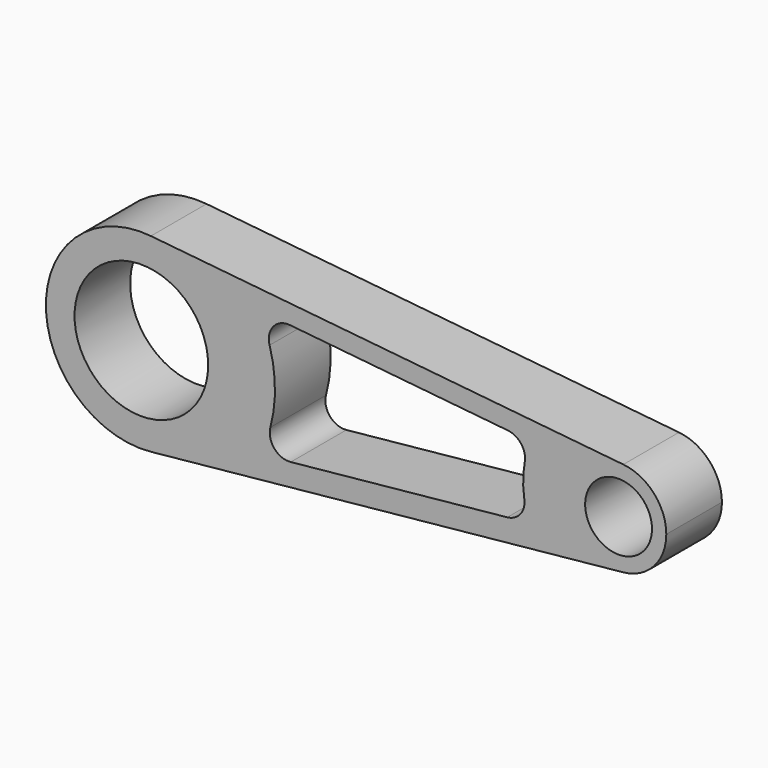
from build123d import *

# Parameters (mm, degrees)
F0_R     = 22.225
F0_R_2   = 11.1125
F1_DEPTH = 23.1302697212


# Not quite as in the source:
# - a feature of the source that left no trace in its solid (it failed there, or was rolled back) is left out


with BuildPart() as f1:
    # F0 (on Front) → F1 (new body)
    with BuildSketch(Plane.XZ):
        with BuildLine():
            ThreePointArc((3.175, 31.5908511281), (23.5464301965, 21.2985474857), (31.75, 0))
            ThreePointArc((31.75, 0), (23.5464301965, -21.2985474857), (3.175, -31.5908511281))
            Line((3.175, -31.5908511281), (160.3375, -15.7954255641))
            ThreePointArc((160.3375, -15.7954255641), (142.875, 0), (160.3375, 15.7954255641))
            Line((160.3375, 15.7954255641), (3.175, 31.5908511281))
        make_face()
        with BuildLine():
            ThreePointArc((42.9352789855, -11.5049692931), (44.4472073469, 0.4982560178), (42.6665789099, 12.4645715579))
            ThreePointArc((42.6665789099, 12.4645715579), (43.8780302599, 18.3037033525), (49.3968044685, 20.5633948632))
            Line((49.3968044685, 20.5633948632), (121.9253365113, 13.2740031244))
            ThreePointArc((121.9253365113, 13.2740031244), (126.3702809224, 10.7659070162), (127.5336137594, 5.7965274156))
            ThreePointArc((127.5336137594, 5.7965274156), (127.0030897981, 0.4429363765), (127.3840485491, -4.9233717695))
            ThreePointArc((127.3840485491, -4.9233717695), (126.1371549085, -9.7886185026), (121.7458582589, -12.226216349))
            Line((121.7458582589, -12.226216349), (49.7038902692, -19.4667065606))
            ThreePointArc((49.7038902692, -19.4667065606), (44.2309158386, -17.261504048), (42.9352789855, -11.5049692931))
        make_face(mode=Mode.SUBTRACT)
        with BuildLine():
            ThreePointArc((3.175, -31.5908511281), (23.5464301965, -21.2985474857), (31.75, 0))
            ThreePointArc((31.75, 0), (23.5464301965, 21.2985474857), (3.175, 31.5908511281))
            ThreePointArc((3.175, 31.5908511281), (-31.75, 0), (3.175, -31.5908511281))
        make_face()
        Circle(F0_R, mode=Mode.SUBTRACT)
        with BuildLine():
            ThreePointArc((174.625, 0), (170.5232150983, 10.6492737428), (160.3375, 15.7954255641))
            ThreePointArc((160.3375, 15.7954255641), (142.875, 0), (160.3375, -15.7954255641))
            ThreePointArc((160.3375, -15.7954255641), (170.5232150983, -10.6492737428), (174.625, 0))
        make_face()
        with Locations((158.75, 0)):
            Circle(F0_R_2, mode=Mode.SUBTRACT)
    extrude(amount=F1_DEPTH)


solid = f1.part
